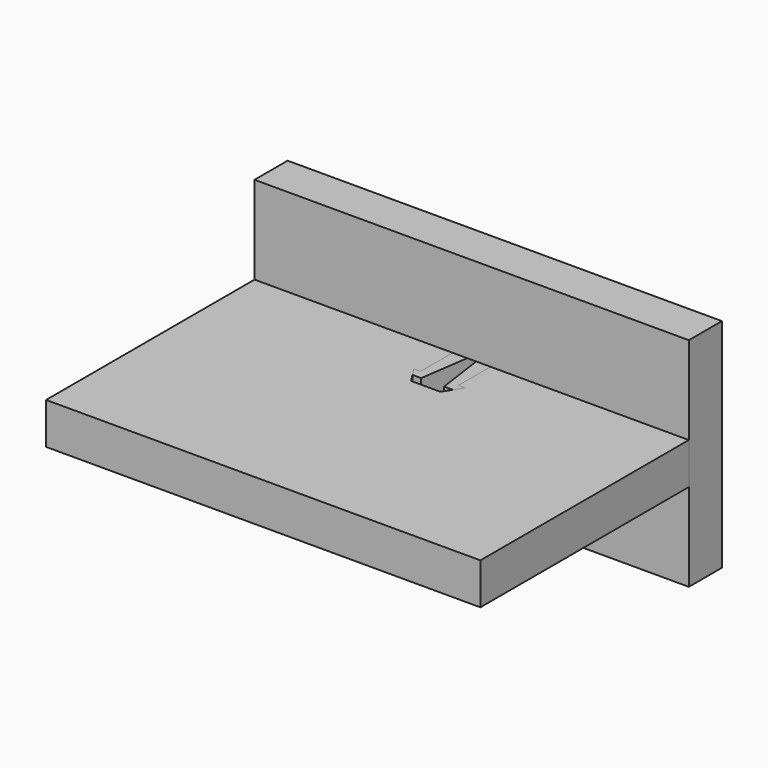
from build123d import *

# Parameters (mm, degrees)
F2_DEPTH = 2.38125
F3_W     = 50
F3_H     = 25
F3_W_2   = 9.1181
F3_H_2   = 4.7625
F4_DEPTH = 4.7625
F6_DEPTH = 2.38125


# Not quite as in the source:
# - a length typed as a fraction of an inch, garbled in the dataset ("3 / 203.2 mm" for 3/8 in), is restored


with BuildPart() as f2:
    # F1 (on Top) → F2 (new body, symmetric)
    with BuildSketch(Plane.XY):
        Polygon((-4.55905, 0), (-25, 0), (-25, -30), (0, -30), (25, -30), (25, 0), (4.55905, 0), (4.55905, 2.38125), (2.1778, 2.38125), (2.1778, -4.61875), (2.97895, -4.61875), (1.6778, -6.61875), (-1.6778, -6.61875), (-2.97895, -4.61875), (-2.1778, -4.61875), (-2.1778, 2.38125), (-4.55905, 2.38125), align=None)
    extrude(amount=F2_DEPTH, both=True)


with BuildPart() as f4:
    # F3 (on Front) → F4 (new body)
    with BuildSketch(Plane.XZ):
        Rectangle(F3_W, F3_H)
        Rectangle(F3_W_2, F3_H_2, mode=Mode.SUBTRACT)
    extrude(amount=-F4_DEPTH)


with BuildPart() as f6:
    # F5 (on Top) → F6 (new body, symmetric)
    with BuildSketch(Plane.XY):
        with BuildLine():
            Line((2.97895, -4.61875), (2.1778, -4.61875))
            Line((2.1778, -4.61875), (2.1778, 2.38125))
            Line((2.1778, 2.38125), (4.55905, 2.38125))
            Line((4.55905, 2.38125), (4.55905, 4.7625))
            Line((4.55905, 4.7625), (10, 4.7625))
            Line((10, 4.7625), (10, 7.14375))
            Line((10, 7.14375), (0, 7.14375))
            Line((0, 7.14375), (0, 2.5338832274))
            ThreePointArc((0, 2.5338832274), (0.1164864538, 2.4904102391), (0.1760098678, 2.38125))
            Line((0.1760098678, 2.38125), (1.3198899433, -5.61875))
            Line((1.3198899433, -5.61875), (2.328375, -5.61875))
            Line((2.328375, -5.61875), (2.97895, -4.61875))
        make_face()
    extrude(amount=F6_DEPTH, both=True)

    # F7: F6 across face


with BuildPart() as f6_1:
    add(f6.part)
    add(f6.part.mirror(Plane(origin=(0, 4.8388166137, 0), x_dir=(0, -1, 0), z_dir=(-1, 0, 0))))


solid = Compound([f2.part, f4.part, f6_1.part])
